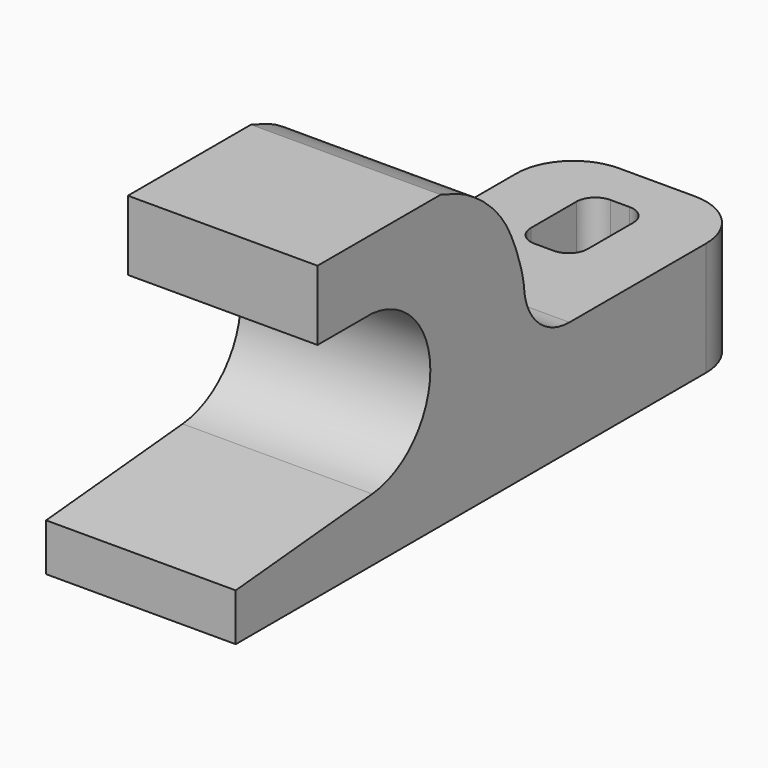
from build123d import *

# Parameters (mm, degrees)
F1_DEPTH    = 10
F2_T1_DEPTH = 10
F2_T3_DEPTH = 21
F2_T5_DEPTH = 21
F3_W        = 3
F3_H        = 5
F4_DEPTH    = 25
F5_R        = 1


# Not quite as in the source:
# - a fillet or chamfer that OpenCascade refuses, or shapes differently, is made with other operations: its cross-section is extruded or revolved along the edge and cut away or added


with BuildPart() as f1:
    # F0 (on Right) → F1 (new body)
    with BuildSketch(Plane.YZ):
        with BuildLine():
            Line((0, 2.5), (0, 0))
            Line((0, 0), (34, 0))
            Line((34, 0), (34, 6))
            Line((34, 6), (19, 6))
            Line((19, 6), (19, 8.927215822))
            add(Edge.make_bspline(
                [(13.5019160807, 15.3781203553), (14.3536763756, 15.0835294533), (15.3076259705, 14.7454615797), (17.8235832578, 12.8012966962), (18.7947445626, 9.9588259689), (18.9257892428, 9.3615105358), (19, 8.927215822)],
                knots=[0, 0, 0, 0, 0.0707143844, 0.1572524963, 0.2414371446, 0.2933722159, 0.2933722159, 0.2933722159, 0.2933722159], degree=3))
            Line((13.5019160807, 15.3781203553), (5.3910082206, 15.3781203553))
            Line((5.3910082206, 15.3781203553), (5.3910082206, 13.2812492201))
            Line((5.3910082206, 13.2812492201), (5.3910082206, 11.7001235485))
            Line((5.3910082206, 11.7001235485), (9, 11.7001235485))
            ThreePointArc((9, 11.7001235485), (12.8276697655, 7.5089175953), (9, 3.317711642))
            Line((9, 3.317711642), (0, 2.5))
        make_face()
    extrude(amount=F1_DEPTH)

    # F2: fillet of radius 3 on 3 edges, made by hand

    # F2_s2 → F2_t1 (join)
    with BuildSketch(Plane.YZ):
        with BuildLine():
            ThreePointArc((19, 8.927215822), (19.9036876994, 6.8531007786), (21.9991169473, 6))
            Line((21.9991169473, 6), (19, 6))
            Line((19, 6), (19, 8.927215822))
        make_face()
    extrude(amount=F2_T1_DEPTH)

    # F2_s4 → F2_t3 (cut)
    with BuildSketch(Plane.XY.offset(-7.5)):
        with BuildLine():
            ThreePointArc((10, 31), (9.1213203436, 33.1213203436), (7, 34))
            Line((7, 34), (10, 34))
            Line((10, 34), (10, 31))
        make_face()
    extrude(amount=F2_T3_DEPTH, mode=Mode.SUBTRACT)

    # F2_s6 → F2_t5 (cut)
    with BuildSketch(Plane.XY.offset(-7.5)):
        with BuildLine():
            ThreePointArc((0, 31), (0.8786796564, 33.1213203436), (3, 34))
            Line((3, 34), (0, 34))
            Line((0, 34), (0, 31))
        make_face()
    extrude(amount=F2_T5_DEPTH, mode=Mode.SUBTRACT)

    # F3 (on face) → F4 (cut)
    with BuildSketch(Plane.XY.offset(6)):
        with Locations((5, 29.0757007897)):
            Rectangle(F3_W, F3_H)
    extrude(amount=-F4_DEPTH, mode=Mode.SUBTRACT)

    # F5
    f5_edges = [f1.edges().sort_by_distance(p)[0] for p in [
        (3.5, 26.575701, 3),
        (3.5, 31.575701, 3),
        (6.5, 26.575701, 3),
        (6.5, 31.575701, 3),
    ]]
    fillet(f5_edges, radius=F5_R)


solid = f1.part
